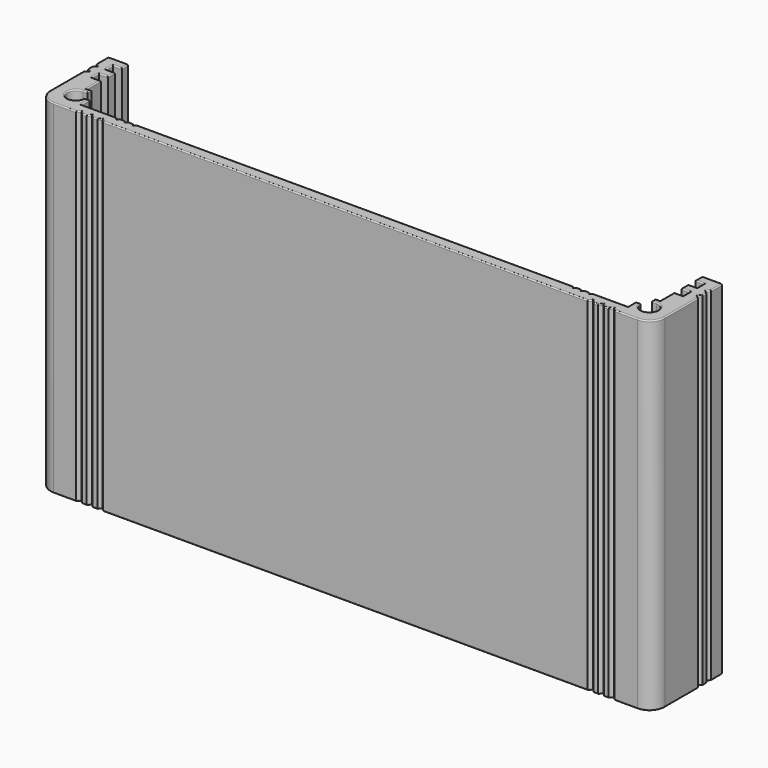
from build123d import *

# Parameters (mm, degrees)
F1_DEPTH     = 58.7
F2_R         = 0.2
F3_R         = 0.2
F4_T1_DEPTH  = 58.7
F4_T4_ANGLE  = 90
F4_T6_ANGLE  = 90
F4_T8_ANGLE  = 90
F4_T10_ANGLE = 90
F4_T12_ANGLE = 90
F4_T14_ANGLE = 90
F4_T16_ANGLE = 90
F4_T18_ANGLE = 90
F5_T1_DEPTH  = 58.7
F5_T4_ANGLE  = 90
F5_T6_ANGLE  = 90
F5_T8_ANGLE  = 90
F5_T10_ANGLE = 90


# Not quite as in the source:
# - a fillet or chamfer that OpenCascade refuses, or shapes differently, is made with other operations: its cross-section is extruded or revolved along the edge and cut away or added


with BuildPart() as f1:
    # F0 (on Top) → F1 (new body)
    with BuildSketch(Plane.XY):
        with BuildLine():
            Line((-52.5, -5.3), (-52.5, -15))
            Line((-52.5, -15), (-46, -15))
            Line((-46, -15), (-45.5, -14.5))
            Line((-45.5, -14.5), (-45, -15))
            Line((-45, -15), (-44.2, -15))
            Line((-44.2, -15), (-43.7, -14.5))
            Line((-43.7, -14.5), (-43.2, -15))
            Line((-43.2, -15), (-42.4, -15))
            Line((-42.4, -15), (-41.9, -14.5))
            Line((-41.9, -14.5), (-41.4, -15))
            Line((-41.4, -15), (0, -15))
            Line((0, -15), (41.4, -15))
            Line((41.4, -15), (41.9, -14.5))
            Line((41.9, -14.5), (42.4, -15))
            Line((42.4, -15), (43.2, -15))
            Line((43.2, -15), (43.7, -14.5))
            Line((43.7, -14.5), (44.2, -15))
            Line((44.2, -15), (45, -15))
            Line((45, -15), (45.5, -14.5))
            Line((45.5, -14.5), (46, -15))
            Line((46, -15), (52.5, -15))
            Line((52.5, -15), (52.5, -5.3))
            Line((52.5, -5.3), (52, -4.8))
            Line((52, -4.8), (52.5, -4.3))
            Line((52.5, -4.3), (52.5, -3.5))
            Line((52.5, -3.5), (52, -3))
            Line((52, -3), (52.5, -2.5))
            Line((52.5, -2.5), (52.5, 0))
            Line((52.5, 0), (49, 0))
            Line((49, 0), (49, -1.5))
            Line((49, -1.5), (50.5, -1.5))
            Line((50.5, -1.5), (50.5, -3))
            Line((50.5, -3), (49, -3))
            Line((49, -3), (49, -4.5))
            Line((49, -4.5), (50.5, -4.5))
            Line((50.5, -4.5), (50.5, -6))
            Line((50.5, -6), (49, -6))
            Line((49, -6), (49, -9))
            Line((49, -9), (48.2, -9))
            Line((48.2, -9), (48.2, -9.8))
            Line((48.2, -9.8), (49, -9.8))
            ThreePointArc((49, -9.8), (50.0606601718, -12.3606601718), (47.5, -11.3))
            Line((47.5, -11.3), (46.7, -11.3))
            Line((46.7, -11.3), (46.7, -13))
            Line((46.7, -13), (40.7, -13))
            Line((40.7, -13), (40.4, -13.3))
            Line((40.4, -13.3), (40.1, -13))
            Line((40.1, -13), (39.3, -13))
            Line((39.3, -13), (39, -13.3))
            Line((39, -13.3), (38.7, -13))
            Line((38.7, -13), (37.9, -13))
            Line((37.9, -13), (37.6, -13.3))
            Line((37.6, -13.3), (37.3, -13))
            Line((37.3, -13), (0, -13))
            Line((0, -13), (-37.3, -13))
            Line((-37.3, -13), (-37.6, -13.3))
            Line((-37.6, -13.3), (-37.9, -13))
            Line((-37.9, -13), (-38.7, -13))
            Line((-38.7, -13), (-39, -13.3))
            Line((-39, -13.3), (-39.3, -13))
            Line((-39.3, -13), (-40.1, -13))
            Line((-40.1, -13), (-40.4, -13.3))
            Line((-40.4, -13.3), (-40.7, -13))
            Line((-40.7, -13), (-46.7, -13))
            Line((-46.7, -13), (-46.7, -11.3))
            Line((-46.7, -11.3), (-47.5, -11.3))
            ThreePointArc((-47.5, -11.3), (-50.0606601718, -12.3606601718), (-49, -9.8))
            Line((-49, -9.8), (-48.2, -9.8))
            Line((-48.2, -9.8), (-48.2, -9))
            Line((-48.2, -9), (-49, -9))
            Line((-49, -9), (-49, -6))
            Line((-49, -6), (-50.5, -6))
            Line((-50.5, -6), (-50.5, -4.5))
            Line((-50.5, -4.5), (-49, -4.5))
            Line((-49, -4.5), (-49, -3))
            Line((-49, -3), (-50.5, -3))
            Line((-50.5, -3), (-50.5, -1.5))
            Line((-50.5, -1.5), (-49, -1.5))
            Line((-49, -1.5), (-49, 0))
            Line((-49, 0), (-52.5, 0))
            Line((-52.5, 0), (-52.5, -2.5))
            Line((-52.5, -2.5), (-52, -3))
            Line((-52, -3), (-52.5, -3.5))
            Line((-52.5, -3.5), (-52.5, -4.3))
            Line((-52.5, -4.3), (-52, -4.8))
            Line((-52, -4.8), (-52.5, -5.3))
        make_face()
    extrude(amount=F1_DEPTH)

    # F2
    f2_edges = [f1.edges().sort_by_distance(p)[0] for p in [
        (-52.5, -10.15, 58.7),
        (-49.25, -15, 58.7),
        (-45.75, -14.75, 58.7),
        (-45.25, -14.75, 58.7),
        (-44.6, -15, 58.7),
        (-43.95, -14.75, 58.7),
        (-43.45, -14.75, 58.7),
        (-42.8, -15, 58.7),
        (-42.15, -14.75, 58.7),
        (-41.65, -14.75, 58.7),
        (0, -15, 58.7),
        (41.65, -14.75, 58.7),
        (42.15, -14.75, 58.7),
        (42.8, -15, 58.7),
        (43.45, -14.75, 58.7),
        (43.95, -14.75, 58.7),
        (44.6, -15, 58.7),
        (45.25, -14.75, 58.7),
        (45.75, -14.75, 58.7),
        (49.25, -15, 58.7),
        (52.5, -10.15, 58.7),
        (52.25, -5.05, 58.7),
        (52.25, -4.55, 58.7),
        (52.5, -3.9, 58.7),
        (52.25, -3.25, 58.7),
        (52.25, -2.75, 58.7),
        (52.5, -1.25, 58.7),
        (50.75, 0, 58.7),
        (49, -0.75, 58.7),
        (49.75, -1.5, 58.7),
        (50.5, -2.25, 58.7),
        (49.75, -3, 58.7),
        (49, -3.75, 58.7),
        (49.75, -4.5, 58.7),
        (50.5, -5.25, 58.7),
        (49.75, -6, 58.7),
        (49, -7.5, 58.7),
        (48.6, -9, 58.7),
        (48.2, -9.4, 58.7),
        (48.6, -9.8, 58.7),
        (50.06066, -12.36066, 58.7),
        (47.1, -11.3, 58.7),
        (46.7, -12.15, 58.7),
        (43.7, -13, 58.7),
        (40.55, -13.15, 58.7),
        (40.25, -13.15, 58.7),
        (39.7, -13, 58.7),
        (39.15, -13.15, 58.7),
        (38.85, -13.15, 58.7),
        (38.3, -13, 58.7),
        (37.75, -13.15, 58.7),
        (37.45, -13.15, 58.7),
        (0, -13, 58.7),
        (-37.45, -13.15, 58.7),
        (-37.75, -13.15, 58.7),
        (-38.3, -13, 58.7),
        (-38.85, -13.15, 58.7),
        (-39.15, -13.15, 58.7),
        (-39.7, -13, 58.7),
        (-40.25, -13.15, 58.7),
        (-40.55, -13.15, 58.7),
        (-43.7, -13, 58.7),
        (-46.7, -12.15, 58.7),
        (-47.1, -11.3, 58.7),
        (-50.06066, -12.36066, 58.7),
        (-48.6, -9.8, 58.7),
        (-48.2, -9.4, 58.7),
        (-48.6, -9, 58.7),
        (-49, -7.5, 58.7),
        (-49.75, -6, 58.7),
        (-50.5, -5.25, 58.7),
        (-49.75, -4.5, 58.7),
        (-49, -3.75, 58.7),
        (-49.75, -3, 58.7),
        (-50.5, -2.25, 58.7),
        (-49.75, -1.5, 58.7),
        (-49, -0.75, 58.7),
        (-50.75, 0, 58.7),
        (-52.5, -1.25, 58.7),
        (-52.25, -2.75, 58.7),
        (-52.25, -3.25, 58.7),
        (-52.5, -3.9, 58.7),
        (-52.25, -4.55, 58.7),
        (-52.25, -5.05, 58.7),
    ]]
    fillet(f2_edges, radius=F2_R)

    # F3
    f3_edges = [f1.edges().sort_by_distance(p)[0] for p in [
        (-52.5, -10.15, 0),
        (-49.25, -15, 0),
        (-45.75, -14.75, 0),
        (-45.25, -14.75, 0),
        (-44.6, -15, 0),
        (-43.95, -14.75, 0),
        (-43.45, -14.75, 0),
        (-42.8, -15, 0),
        (-42.15, -14.75, 0),
        (-41.65, -14.75, 0),
        (0, -15, 0),
        (41.65, -14.75, 0),
        (42.15, -14.75, 0),
        (42.8, -15, 0),
        (43.45, -14.75, 0),
        (43.95, -14.75, 0),
        (44.6, -15, 0),
        (45.25, -14.75, 0),
        (45.75, -14.75, 0),
        (49.25, -15, 0),
        (52.5, -10.15, 0),
        (52.25, -5.05, 0),
        (52.25, -4.55, 0),
        (52.5, -3.9, 0),
        (52.25, -3.25, 0),
        (52.25, -2.75, 0),
        (52.5, -1.25, 0),
        (50.75, 0, 0),
        (49, -0.75, 0),
        (49.75, -1.5, 0),
        (50.5, -2.25, 0),
        (49.75, -3, 0),
        (49, -3.75, 0),
        (49.75, -4.5, 0),
        (50.5, -5.25, 0),
        (49.75, -6, 0),
        (49, -7.5, 0),
        (48.6, -9, 0),
        (48.2, -9.4, 0),
        (48.6, -9.8, 0),
        (50.06066, -12.36066, 0),
        (47.1, -11.3, 0),
        (46.7, -12.15, 0),
        (43.7, -13, 0),
        (40.55, -13.15, 0),
        (40.25, -13.15, 0),
        (39.7, -13, 0),
        (39.15, -13.15, 0),
        (38.85, -13.15, 0),
        (38.3, -13, 0),
        (37.75, -13.15, 0),
        (37.45, -13.15, 0),
        (0, -13, 0),
        (-37.45, -13.15, 0),
        (-37.75, -13.15, 0),
        (-38.3, -13, 0),
        (-38.85, -13.15, 0),
        (-39.15, -13.15, 0),
        (-39.7, -13, 0),
        (-40.25, -13.15, 0),
        (-40.55, -13.15, 0),
        (-43.7, -13, 0),
        (-46.7, -12.15, 0),
        (-47.1, -11.3, 0),
        (-50.06066, -12.36066, 0),
        (-48.6, -9.8, 0),
        (-48.2, -9.4, 0),
        (-48.6, -9, 0),
        (-49, -7.5, 0),
        (-49.75, -6, 0),
        (-50.5, -5.25, 0),
        (-49.75, -4.5, 0),
        (-49, -3.75, 0),
        (-49.75, -3, 0),
        (-50.5, -2.25, 0),
        (-49.75, -1.5, 0),
        (-49, -0.75, 0),
        (-50.75, 0, 0),
        (-52.5, -1.25, 0),
        (-52.25, -2.75, 0),
        (-52.25, -3.25, 0),
        (-52.5, -3.9, 0),
        (-52.25, -4.55, 0),
        (-52.25, -5.05, 0),
    ]]
    fillet(f3_edges, radius=F3_R)

    # F4: fillet of radius 0.3 on 4 edges, made by hand

    # F4_s2 → F4_t1 (cut)
    with BuildSketch(Plane.XY):
        with BuildLine():
            ThreePointArc((-52.5, -0.3), (-52.4121320344, -0.0878679656), (-52.2, 0))
            Line((-52.2, 0), (-52.5, 0))
            Line((-52.5, 0), (-52.5, -0.3))
        make_face()
        with BuildLine():
            ThreePointArc((-49.3, 0), (-49.0878679656, -0.0878679656), (-49, -0.3))
            Line((-49, -0.3), (-49, 0))
            Line((-49, 0), (-49.3, 0))
        make_face()
        with BuildLine():
            ThreePointArc((49.3, 0), (49.0878679656, -0.0878679656), (49, -0.3))
            Line((49, -0.3), (49, 0))
            Line((49, 0), (49.3, 0))
        make_face()
        with BuildLine():
            ThreePointArc((52.5, -0.3), (52.4121320344, -0.0878679656), (52.2, 0))
            Line((52.2, 0), (52.5, 0))
            Line((52.5, 0), (52.5, -0.3))
        make_face()
    extrude(amount=F4_T1_DEPTH, mode=Mode.SUBTRACT)

    # F4_s3 → F4_t4 (revolve, cut)
    with BuildSketch(Plane.YZ.offset(52.2)):
        with BuildLine():
            ThreePointArc((-0.2, 0), (-0.0585786438, 0.0585786438), (0, 0.2))
            Line((0, 0.2), (0, 0))
            Line((0, 0), (-0.2, 0))
        make_face()
    revolve(axis=Axis((52.2, -0.3, 0), (0, 0, -1)), revolution_arc=F4_T4_ANGLE, mode=Mode.SUBTRACT)

    # F4_s5 → F4_t6 (revolve, cut)
    with BuildSketch(Plane.XZ.offset(0.3)):
        with BuildLine():
            ThreePointArc((52.3, 58.7), (52.4414213562, 58.6414213562), (52.5, 58.5))
            Line((52.5, 58.5), (52.5, 58.7))
            Line((52.5, 58.7), (52.3, 58.7))
        make_face()
    revolve(axis=Axis((52.2, -0.3, 58.7), (0, 0, 1)), revolution_arc=F4_T6_ANGLE, mode=Mode.SUBTRACT)

    # F4_s7 → F4_t8 (revolve, cut)
    with BuildSketch(Plane.XZ.offset(0.3)):
        with BuildLine():
            ThreePointArc((49.2, 0), (49.0585786438, 0.0585786438), (49, 0.2))
            Line((49, 0.2), (49, 0))
            Line((49, 0), (49.2, 0))
        make_face()
    revolve(axis=Axis((49.3, -0.3, 0), (0, 0, -1)), revolution_arc=F4_T8_ANGLE, mode=Mode.SUBTRACT)

    # F4_s9 → F4_t10 (revolve, cut)
    with BuildSketch(Plane.YZ.offset(49.3)):
        with BuildLine():
            ThreePointArc((-0.2, 58.7), (-0.0585786438, 58.6414213562), (0, 58.5))
            Line((0, 58.5), (0, 58.7))
            Line((0, 58.7), (-0.2, 58.7))
        make_face()
    revolve(axis=Axis((49.3, -0.3, 58.7), (0, 0, 1)), revolution_arc=F4_T10_ANGLE, mode=Mode.SUBTRACT)

    # F4_s11 → F4_t12 (revolve, cut)
    with BuildSketch(Plane.YZ.offset(-49.3)):
        with BuildLine():
            ThreePointArc((-0.2, 0), (-0.0585786438, 0.0585786438), (0, 0.2))
            Line((0, 0.2), (0, 0))
            Line((0, 0), (-0.2, 0))
        make_face()
    revolve(axis=Axis((-49.3, -0.3, 0), (0, 0, -1)), revolution_arc=F4_T12_ANGLE, mode=Mode.SUBTRACT)

    # F4_s13 → F4_t14 (revolve, cut)
    with BuildSketch(Plane.XZ.offset(0.3)):
        with BuildLine():
            ThreePointArc((-49.2, 58.7), (-49.0585786438, 58.6414213562), (-49, 58.5))
            Line((-49, 58.5), (-49, 58.7))
            Line((-49, 58.7), (-49.2, 58.7))
        make_face()
    revolve(axis=Axis((-49.3, -0.3, 58.7), (0, 0, 1)), revolution_arc=F4_T14_ANGLE, mode=Mode.SUBTRACT)

    # F4_s15 → F4_t16 (revolve, cut)
    with BuildSketch(Plane.XZ.offset(0.3)):
        with BuildLine():
            ThreePointArc((-52.3, 0), (-52.4414213562, 0.0585786438), (-52.5, 0.2))
            Line((-52.5, 0.2), (-52.5, 0))
            Line((-52.5, 0), (-52.3, 0))
        make_face()
    revolve(axis=Axis((-52.2, -0.3, 0), (0, 0, -1)), revolution_arc=F4_T16_ANGLE, mode=Mode.SUBTRACT)

    # F4_s17 → F4_t18 (revolve, cut)
    with BuildSketch(Plane.YZ.offset(-52.2)):
        with BuildLine():
            ThreePointArc((-0.2, 58.7), (-0.0585786438, 58.6414213562), (0, 58.5))
            Line((0, 58.5), (0, 58.7))
            Line((0, 58.7), (-0.2, 58.7))
        make_face()
    revolve(axis=Axis((-52.2, -0.3, 58.7), (0, 0, 1)), revolution_arc=F4_T18_ANGLE, mode=Mode.SUBTRACT)

    # F5: fillet of radius 2.6 on 2 edges, made by hand

    # F5_s2 → F5_t1 (cut)
    with BuildSketch(Plane.XY):
        with BuildLine():
            ThreePointArc((-52.5, -12.4), (-51.7384776311, -14.2384776311), (-49.9, -15))
            Line((-49.9, -15), (-52.5, -15))
            Line((-52.5, -15), (-52.5, -12.4))
        make_face()
        with BuildLine():
            ThreePointArc((52.5, -12.4), (51.7384776311, -14.2384776311), (49.9, -15))
            Line((49.9, -15), (52.5, -15))
            Line((52.5, -15), (52.5, -12.4))
        make_face()
    extrude(amount=F5_T1_DEPTH, mode=Mode.SUBTRACT)

    # F5_s3 → F5_t4 (revolve, cut)
    with BuildSketch(Plane.XZ.offset(12.4)):
        with BuildLine():
            ThreePointArc((52.3, 0), (52.4414213562, 0.0585786438), (52.5, 0.2))
            Line((52.5, 0.2), (52.5, 0))
            Line((52.5, 0), (52.3, 0))
        make_face()
    revolve(axis=Axis((49.9, -12.4, 0), (0, 0, -1)), revolution_arc=F5_T4_ANGLE, mode=Mode.SUBTRACT)

    # F5_s5 → F5_t6 (revolve, cut)
    with BuildSketch(Plane.YZ.offset(49.9)):
        with BuildLine():
            ThreePointArc((-14.8, 58.7), (-14.9414213562, 58.6414213562), (-15, 58.5))
            Line((-15, 58.5), (-15, 58.7))
            Line((-15, 58.7), (-14.8, 58.7))
        make_face()
    revolve(axis=Axis((49.9, -12.4, 58.7), (0, 0, 1)), revolution_arc=F5_T6_ANGLE, mode=Mode.SUBTRACT)

    # F5_s7 → F5_t8 (revolve, cut)
    with BuildSketch(Plane.YZ.offset(-49.9)):
        with BuildLine():
            ThreePointArc((-14.8, 0), (-14.9414213562, 0.0585786438), (-15, 0.2))
            Line((-15, 0.2), (-15, 0))
            Line((-15, 0), (-14.8, 0))
        make_face()
    revolve(axis=Axis((-49.9, -12.4, 0), (0, 0, -1)), revolution_arc=F5_T8_ANGLE, mode=Mode.SUBTRACT)

    # F5_s9 → F5_t10 (revolve, cut)
    with BuildSketch(Plane.XZ.offset(12.4)):
        with BuildLine():
            ThreePointArc((-52.3, 58.7), (-52.4414213562, 58.6414213562), (-52.5, 58.5))
            Line((-52.5, 58.5), (-52.5, 58.7))
            Line((-52.5, 58.7), (-52.3, 58.7))
        make_face()
    revolve(axis=Axis((-49.9, -12.4, 58.7), (0, 0, 1)), revolution_arc=F5_T10_ANGLE, mode=Mode.SUBTRACT)


solid = f1.part
